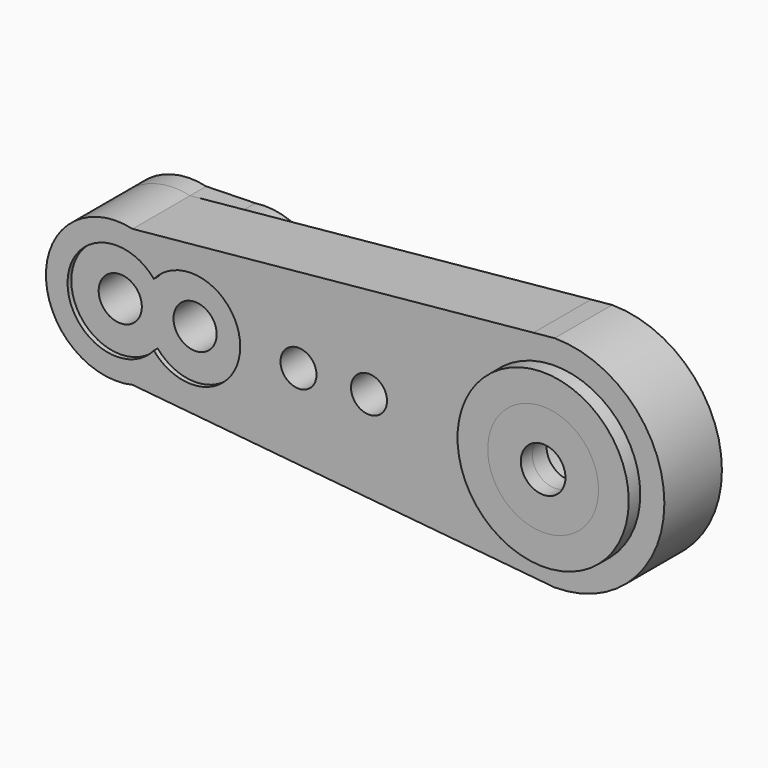
from build123d import *
from build123d import SkipClean  # not in build123d's __all__

# Parameters (mm, degrees)
F0_R     = 1.5
F0_R_2   = 1.25
F0_R_3   = 1.55
F1_DEPTH = 5
F2_R     = 1.5
F3_DEPTH = 0.33
F2_R_2   = 5.95
F2_R_3   = 3.85
F4_DEPTH = 1
F5_R     = 1.5
F6_DEPTH = 1.4
F5_R_2   = 5.675
F5_R_3   = 4.4
F7_DEPTH = 1.5
F5_R_4   = 1.55
F8_DEPTH = 3.77
F2_R_4   = 1.55
F9_DEPTH = 1


# Not quite as in the source:
# - after a boolean that leaves OpenCascade's solid faulty, fix() repairs it


with BuildPart() as f1:
    # F0 (on Front) → F1 (new body)
    with BuildSketch(Plane.XZ):
        with BuildLine():
            Line((-29.334043409, -4.7712305422), (-1.4696901505, -7.4820208408))
            Line((-1.4696901505, -7.4820208408), (0, -7.625))
            ThreePointArc((0, -7.625), (7.625, 0), (0, 7.625))
            Line((0, 7.625), (-1.4696901505, 7.4820208408))
            Line((-1.4696901505, 7.4820208408), (-29.334043409, 4.7712305422))
            ThreePointArc((-29.334043409, 4.7712305422), (-35.35, 0), (-29.334043409, -4.7712305422))
        make_face()
        with Locations((-30.45, 0)):
            Circle(F0_R, mode=Mode.SUBTRACT)
        with Locations((-25.25, 0)):
            Circle(F0_R, mode=Mode.SUBTRACT)
        with Locations((-17.8, 0)):
            Circle(F0_R_2, mode=Mode.SUBTRACT)
        with Locations((-12.9, 0)):
            Circle(F0_R_2, mode=Mode.SUBTRACT)
        Circle(F0_R_3, mode=Mode.SUBTRACT)
    extrude(amount=F1_DEPTH)

    # F2 (on face) → F3 (cut)
    with BuildSketch(Plane.XZ.offset(5)):
        with BuildLine():
            ThreePointArc((-27.85, -2.19089023), (-28.65, 0), (-27.85, 2.19089023))
            ThreePointArc((-27.85, 2.19089023), (-33.85, 0), (-27.85, -2.19089023))
        make_face()
        with Locations((-30.45, 0)):
            Circle(F2_R, mode=Mode.SUBTRACT)
        with BuildLine():
            ThreePointArc((-27.85, -2.19089023), (-27.2562561155, -1.166190379), (-27.05, 0))
            ThreePointArc((-27.05, 0), (-27.2562561155, 1.166190379), (-27.85, 2.19089023))
            ThreePointArc((-27.85, 2.19089023), (-28.65, 0), (-27.85, -2.19089023))
        make_face()
        with BuildLine():
            ThreePointArc((-27.85, 2.19089023), (-27.2562561155, 1.166190379), (-27.05, 0))
            ThreePointArc((-27.05, 0), (-27.2562561155, -1.166190379), (-27.85, -2.19089023))
            ThreePointArc((-27.85, -2.19089023), (-24.083809621, -3.1937438845), (-21.85, 0))
            ThreePointArc((-21.85, 0), (-24.083809621, 3.1937438845), (-27.85, 2.19089023))
        make_face()
        with Locations((-25.25, 0)):
            Circle(F2_R, mode=Mode.SUBTRACT)
    extrude(amount=-F3_DEPTH, mode=Mode.SUBTRACT)

    # F2 (on face) → F4 (join)
    with BuildSketch(Plane.XZ.offset(5)):
        Circle(F2_R_2)
        Circle(F2_R_3, mode=Mode.SUBTRACT)
    extrude(amount=F4_DEPTH)

    # F5 (on face) → F6 (join)
    with BuildSketch(Plane(origin=(0, 0, 0), x_dir=(-1, 0, 0), z_dir=(0, 1, 0))):
        with BuildLine():
            ThreePointArc((25.9187577076, -4.8541490633), (26.9215224824, -4.6060843013), (27.85, -4.1533119315))
            ThreePointArc((27.85, -4.1533119315), (28.5665087739, -4.5235451585), (29.334043409, -4.7712305422))
            ThreePointArc((29.334043409, -4.7712305422), (35.35, 0), (29.334043409, 4.7712305422))
            ThreePointArc((29.334043409, 4.7712305422), (28.5665087739, 4.5235451585), (27.85, 4.1533119315))
            ThreePointArc((27.85, 4.1533119315), (26.9215224824, 4.6060843013), (25.9187577076, 4.8541490633))
            ThreePointArc((25.9187577076, 4.8541490633), (20.35, 0), (25.9187577076, -4.8541490633))
        make_face()
        with Locations((25.25, 0)):
            Circle(F5_R, mode=Mode.SUBTRACT)
        with Locations((30.45, 0)):
            Circle(F5_R, mode=Mode.SUBTRACT)
        with BuildLine():
            ThreePointArc((29.334043409, -4.7712305422), (28.5665087739, -4.5235451585), (27.85, -4.1533119315))
            ThreePointArc((27.85, -4.1533119315), (26.9215224824, -4.6060843013), (25.9187577076, -4.8541490633))
            Line((25.9187577076, -4.8541490633), (29.334043409, -4.7712305422))
        make_face()
        with BuildLine():
            ThreePointArc((27.85, 4.1533119315), (28.5665087739, 4.5235451585), (29.334043409, 4.7712305422))
            Line((29.334043409, 4.7712305422), (25.9187577076, 4.8541490633))
            ThreePointArc((25.9187577076, 4.8541490633), (26.9215224824, 4.6060843013), (27.85, 4.1533119315))
        make_face()
    with SkipClean():  # cleaning this boolean's faces spoils the solid; the shape is the same uncleaned
        extrude(amount=F6_DEPTH)

    # F5 (on face) → F7 (join)
    with BuildSketch(Plane(origin=(0, 0, 0), x_dir=(-1, 0, 0), z_dir=(0, 1, 0))):
        Circle(F5_R_2)
        Circle(F5_R_3, mode=Mode.SUBTRACT)
    extrude(amount=F7_DEPTH)

    add(f1.part.fix(), mode=Mode.REPLACE)

    # F5 (on face) → F8 (cut)
    with BuildSketch(Plane(origin=(0, 0, 0), x_dir=(-1, 0, 0), z_dir=(0, 1, 0))):
        Circle(F5_R_3)
        Circle(F5_R_4, mode=Mode.SUBTRACT)
    extrude(amount=-F8_DEPTH, mode=Mode.SUBTRACT)


with BuildPart() as f9:
    # F2 (on face) → F9 (new body)
    with BuildSketch(Plane.XZ.offset(5)):
        Circle(F2_R_3)
        Circle(F2_R_4, mode=Mode.SUBTRACT)
    extrude(amount=F9_DEPTH)


solid = Compound([f1.part, f9.part])
